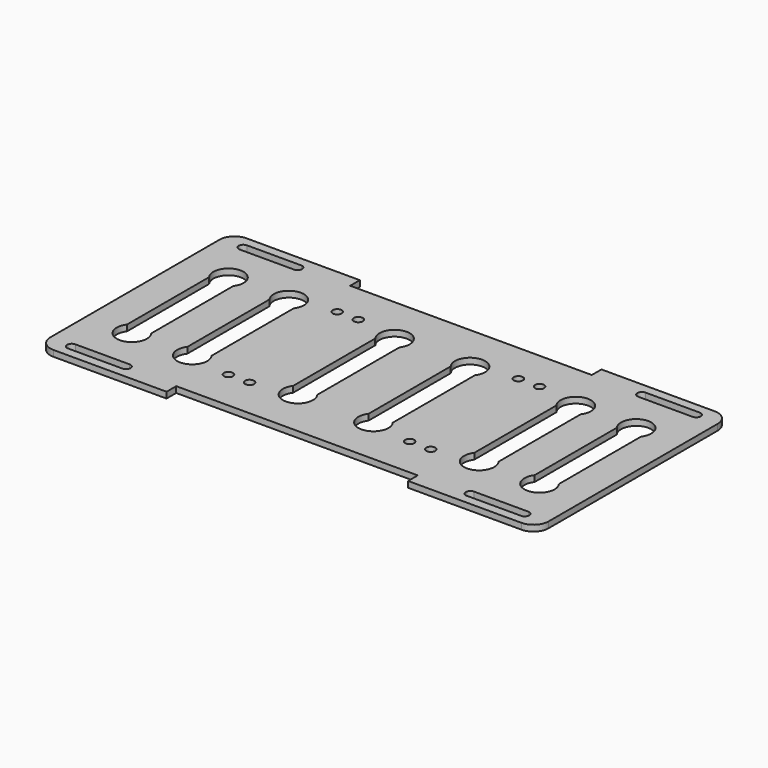
from build123d import *

# Parameters (mm, degrees)
F0_W      = 165
F0_H      = 80
F1_DEPTH  = 2
F2_W      = 21
F2_H      = 3
F3_DEPTH  = 2
F4_R      = 1.49999
F5_W      = 165
F5_H      = 80
F5_R      = 1.5
F6_DEPTH  = 2
F7_DEPTH  = 2
F8_R      = 5
F9_R      = 5
F11_DEPTH = 2.001
F12_W     = 80
F12_H     = 8
F13_DEPTH = 2.001


# Not quite as in the source:
# - a fillet or chamfer is up to 0.001 mm smaller than in the source, because OpenCascade refuses the exact size
# - ends of sketch curves that miss each other by under 0.0002 mm in the source are joined


with BuildPart() as f1:
    # F0 (on Top) → F1 (new body)
    with BuildSketch(Plane.XY):
        Rectangle(F0_W, F0_H)
    extrude(amount=F1_DEPTH)

    # F2 (on face) → F3 (cut)
    with BuildSketch(Plane.XY.offset(2)):
        with Locations((-66, 35.5)):
            Rectangle(F2_W, F2_H)
        with Locations((66, 35.5)):
            Rectangle(F2_W, F2_H)
        with Locations((66, -35.5)):
            Rectangle(F2_W, F2_H)
        with Locations((-66, -35.5)):
            Rectangle(F2_W, F2_H)
    extrude(amount=-F3_DEPTH, mode=Mode.SUBTRACT)

    # F4 (radius 1.5 in the source; OpenCascade refuses exactly that, so slightly less here)
    f4_edges = [f1.edges().sort_by_distance(p)[0] for p in [
        (76.5, -37, 1),
        (-55.5, 34, 1),
        (-55.5, -37, 1),
        (76.5, 34, 1),
        (55.5, 37, 1),
        (55.5, -34, 1),
        (-76.5, -34, 1),
        (-76.5, 37, 1),
        (-76.5, 34, 1),
        (-55.5, 37, 1),
        (76.5, 37, 1),
        (55.5, 34, 1),
        (76.5, -34, 1),
        (55.5, -37, 1),
        (-76.5, -37, 1),
        (-55.5, -34, 1),
    ]]
    fillet(f4_edges, radius=F4_R)

    # F5 (on face) → F6 (join)
    with BuildSketch(Plane.XY.offset(2)):
        Rectangle(F5_W, F5_H)
        with BuildLine():
            ThreePointArc((-76.5, -35.49999), (-76.0606631007, -34.4393368993), (-75.00001, -34))
            Line((-75.00001, -34), (-56.99999, -34))
            ThreePointArc((-56.99999, -34), (-55.9393368993, -34.4393368993), (-55.5, -35.49999))
            ThreePointArc((-55.5, -35.49999), (-55.9393368993, -36.5606631007), (-56.99999, -37))
            Line((-56.99999, -37), (-75.00001, -37))
            ThreePointArc((-75.00001, -37), (-76.0606631007, -36.5606631007), (-76.5, -35.49999))
        make_face(mode=Mode.SUBTRACT)
        with Locations((-33.5, -22.5)):
            Circle(F5_R, mode=Mode.SUBTRACT)
        with Locations((-26.5, -22.5)):
            Circle(F5_R, mode=Mode.SUBTRACT)
        with Locations((26.5, -22.5)):
            Circle(F5_R, mode=Mode.SUBTRACT)
        with Locations((33.5, -22.5)):
            Circle(F5_R, mode=Mode.SUBTRACT)
        with BuildLine():
            ThreePointArc((55.5, -35.49999), (55.9393368993, -34.4393368993), (56.99999, -34))
            Line((56.99999, -34), (75.00001, -34))
            ThreePointArc((75.00001, -34), (76.0606631007, -34.4393368993), (76.5, -35.49999))
            ThreePointArc((76.5, -35.49999), (76.0606631007, -36.5606631007), (75.00001, -37))
            Line((75.00001, -37), (56.99999, -37))
            ThreePointArc((56.99999, -37), (55.9393368993, -36.5606631007), (55.5, -35.49999))
        make_face(mode=Mode.SUBTRACT)
        with BuildLine():
            ThreePointArc((-76.5, 35.50001), (-76.0606631007, 36.5606631007), (-75.00001, 37))
            Line((-75.00001, 37), (-56.99999, 37))
            ThreePointArc((-56.99999, 37), (-55.9393368993, 36.5606631007), (-55.5, 35.50001))
            ThreePointArc((-55.5, 35.50001), (-55.9393368993, 34.4393368993), (-56.99999, 34))
            Line((-56.99999, 34), (-75.00001, 34))
            ThreePointArc((-75.00001, 34), (-76.0606631007, 34.4393368993), (-76.5, 35.50001))
        make_face(mode=Mode.SUBTRACT)
        with Locations((-33.5, 22.5)):
            Circle(F5_R, mode=Mode.SUBTRACT)
        with Locations((-26.5, 22.5)):
            Circle(F5_R, mode=Mode.SUBTRACT)
        with Locations((26.5, 22.5)):
            Circle(F5_R, mode=Mode.SUBTRACT)
        with Locations((33.5, 22.5)):
            Circle(F5_R, mode=Mode.SUBTRACT)
        with BuildLine():
            ThreePointArc((55.5, 35.50001), (55.9393368993, 36.5606631007), (56.99999, 37))
            Line((56.99999, 37), (75.00001, 37))
            ThreePointArc((75.00001, 37), (76.0606631007, 36.5606631007), (76.5, 35.50001))
            ThreePointArc((76.5, 35.50001), (76.0606631007, 34.4393368993), (75.00001, 34))
            Line((75.00001, 34), (56.99999, 34))
            ThreePointArc((56.99999, 34), (55.9393368993, 34.4393368993), (55.5, 35.50001))
        make_face(mode=Mode.SUBTRACT)
    extrude(amount=F6_DEPTH)

    # F7 (cut): a face of the model
    f7_faces = [f1.faces().sort_by_distance(p)[0] for p in [
        (0, 0, 0),
    ]]
    extrude(f7_faces, amount=-F7_DEPTH, mode=Mode.SUBTRACT)

    # F8
    f8_edges = [f1.edges().sort_by_distance(p)[0] for p in [
        (82.5, 40, 3),
    ]]
    fillet(f8_edges, radius=F8_R)

    # F9
    f9_edges = [f1.edges().sort_by_distance(p)[0] for p in [
        (82.5, -40, 3),
        (-82.5, -40, 3),
        (-82.5, 40, 3),
    ]]
    fillet(f9_edges, radius=F9_R)

    # F10 (on face) → F11 (cut, through all)
    with BuildSketch(Plane.XY.offset(4)):
        with BuildLine():
            ThreePointArc((-63.5, 17), (-67.5, 15), (-71.5, 17))
            Line((-71.5, 17), (-71.5, -6.31e-08))
            ThreePointArc((-71.5, -6.31e-08), (-67.5000000315, 4), (-63.5, 0))
            Line((-63.5, 0), (-63.5, 17))
        make_face()
        with BuildLine():
            ThreePointArc((-63.5, 0), (-67.4999999685, -4), (-71.5, -6.31e-08))
            Line((-71.5, -6.31e-08), (-71.5, -17))
            ThreePointArc((-71.5, -17), (-67.5, -15), (-63.5, -17))
            Line((-63.5, -17), (-63.5, 0))
        make_face()
        with BuildLine():
            Line((-71.5, -20), (-71.5, -17))
            ThreePointArc((-71.5, -17), (-69.0811388301, -24.7434164903), (-62.5, -20))
            ThreePointArc((-62.5, -20), (-62.7565835097, -18.4188611699), (-63.5, -17))
            Line((-63.5, -17), (-63.5, -20))
            Line((-63.5, -20), (-71.5, -20))
        make_face()
        with BuildLine():
            ThreePointArc((-63.5, -17), (-67.5, -15), (-71.5, -17))
            Line((-71.5, -17), (-71.5, -20))
            Line((-71.5, -20), (-63.5, -20))
            Line((-63.5, -20), (-63.5, -17))
        make_face()
        with BuildLine():
            ThreePointArc((-63.5, 0), (-67.5000000315, 4), (-71.5, -6.31e-08))
            ThreePointArc((-71.5, -6.31e-08), (-67.4999999685, -4), (-63.5, 0))
        make_face()
        with BuildLine():
            Line((-71.5, 20), (-71.5, 17))
            ThreePointArc((-71.5, 17), (-67.5, 15), (-63.5, 17))
            Line((-63.5, 17), (-63.5, 20))
            Line((-63.5, 20), (-71.5, 20))
        make_face()
        with BuildLine():
            ThreePointArc((-63.5, 17), (-62.7565835097, 18.4188611699), (-62.5, 20))
            ThreePointArc((-62.5, 20), (-69.0811388301, 24.7434164903), (-71.5, 17))
            Line((-71.5, 17), (-71.5, 20))
            Line((-71.5, 20), (-63.5, 20))
            Line((-63.5, 20), (-63.5, 17))
        make_face()
        with BuildLine():
            ThreePointArc((-43.5, 17), (-42.7565835097, 18.4188611699), (-42.5, 20))
            ThreePointArc((-42.5, 20), (-49.0811388301, 24.7434164903), (-51.5, 17))
            Line((-51.5, 17), (-51.5, 20))
            Line((-51.5, 20), (-43.5, 20))
            Line((-43.5, 20), (-43.5, 17))
        make_face()
        with BuildLine():
            Line((-51.5, 20), (-51.5, 17))
            ThreePointArc((-51.5, 17), (-47.5, 15), (-43.5, 17))
            Line((-43.5, 17), (-43.5, 20))
            Line((-43.5, 20), (-51.5, 20))
        make_face()
        with BuildLine():
            ThreePointArc((-43.5, 17), (-47.5, 15), (-51.5, 17))
            Line((-51.5, 17), (-51.5, -2.04e-08))
            ThreePointArc((-51.5, -2.04e-08), (-47.5000000102, 4), (-43.5, 0))
            Line((-43.5, 0), (-43.5, 17))
        make_face()
        with BuildLine():
            ThreePointArc((-43.5, 0), (-47.5000000102, 4), (-51.5, -2.04e-08))
            ThreePointArc((-51.5, -2.04e-08), (-47.4999999898, -4), (-43.5, 0))
        make_face()
        with BuildLine():
            ThreePointArc((-43.5, 0), (-47.4999999898, -4), (-51.5, -2.04e-08))
            Line((-51.5, -2.04e-08), (-51.5, -17))
            ThreePointArc((-51.5, -17), (-47.5, -15), (-43.5, -17))
            Line((-43.5, -17), (-43.5, 0))
        make_face()
        with BuildLine():
            ThreePointArc((-43.5, -17), (-47.5, -15), (-51.5, -17))
            Line((-51.5, -17), (-51.5, -20))
            Line((-51.5, -20), (-43.5, -20))
            Line((-43.5, -20), (-43.5, -17))
        make_face()
        with BuildLine():
            Line((-51.5, -20), (-51.5, -17))
            ThreePointArc((-51.5, -17), (-49.0811388301, -24.7434164903), (-42.5, -20))
            ThreePointArc((-42.5, -20), (-42.7565835097, -18.4188611699), (-43.5, -17))
            Line((-43.5, -17), (-43.5, -20))
            Line((-43.5, -20), (-51.5, -20))
        make_face()
        with BuildLine():
            ThreePointArc((-8.5, 17), (-7.7565835097, 18.4188611699), (-7.5, 20))
            ThreePointArc((-7.5, 20), (-14.0811388301, 24.7434164903), (-16.5, 17))
            Line((-16.5, 17), (-16.5, 20))
            Line((-16.5, 20), (-8.5, 20))
            Line((-8.5, 20), (-8.5, 17))
        make_face()
        with BuildLine():
            Line((-16.5, 20), (-16.5, 17))
            ThreePointArc((-16.5, 17), (-12.5, 15), (-8.5, 17))
            Line((-8.5, 17), (-8.5, 20))
            Line((-8.5, 20), (-16.5, 20))
        make_face()
        with BuildLine():
            ThreePointArc((-8.5, 17), (-12.5, 15), (-16.5, 17))
            Line((-16.5, 17), (-16.5, 8.4e-09))
            ThreePointArc((-16.5, 8.4e-09), (-12.4999999958, 4), (-8.5, 0))
            Line((-8.5, 0), (-8.5, 17))
        make_face()
        with BuildLine():
            ThreePointArc((-8.5, 0), (-12.4999999958, 4), (-16.5, 8.4e-09))
            ThreePointArc((-16.5, 8.4e-09), (-12.5000000042, -4), (-8.5, 0))
        make_face()
        with BuildLine():
            ThreePointArc((-8.5, 0), (-12.5000000042, -4), (-16.5, 8.4e-09))
            Line((-16.5, 8.4e-09), (-16.5, -17))
            ThreePointArc((-16.5, -17), (-12.5, -15), (-8.5, -17))
            Line((-8.5, -17), (-8.5, 0))
        make_face()
        with BuildLine():
            ThreePointArc((-8.5, -17), (-12.5, -15), (-16.5, -17))
            Line((-16.5, -17), (-16.5, -20))
            Line((-16.5, -20), (-8.5, -20))
            Line((-8.5, -20), (-8.5, -17))
        make_face()
        with BuildLine():
            Line((-16.5, -20), (-16.5, -17))
            ThreePointArc((-16.5, -17), (-14.0811388301, -24.7434164903), (-7.5, -20))
            ThreePointArc((-7.5, -20), (-7.7565835097, -18.4188611699), (-8.5, -17))
            Line((-8.5, -17), (-8.5, -20))
            Line((-8.5, -20), (-16.5, -20))
        make_face()
        with BuildLine():
            ThreePointArc((16.5, 17), (17.2434164903, 18.4188611699), (17.5, 20))
            ThreePointArc((17.5, 20), (10.9188611699, 24.7434164903), (8.5, 17))
            Line((8.5, 17), (8.5, 20))
            Line((8.5, 20), (16.5, 20))
            Line((16.5, 20), (16.5, 17))
        make_face()
        with BuildLine():
            Line((8.5, 20), (8.5, 17))
            ThreePointArc((8.5, 17), (12.5, 15), (16.5, 17))
            Line((16.5, 17), (16.5, 20))
            Line((16.5, 20), (8.5, 20))
        make_face()
        with BuildLine():
            ThreePointArc((16.5, 17), (12.5, 15), (8.5, 17))
            Line((8.5, 17), (8.5, 8.4e-09))
            ThreePointArc((8.5, 8.4e-09), (12.5000000042, 4), (16.5, 0))
            Line((16.5, 0), (16.5, 17))
        make_face()
        with BuildLine():
            ThreePointArc((16.5, 0), (12.5000000042, 4), (8.5, 8.4e-09))
            ThreePointArc((8.5, 8.4e-09), (12.4999999958, -4), (16.5, 0))
        make_face()
        with BuildLine():
            ThreePointArc((16.5, 0), (12.4999999958, -4), (8.5, 8.4e-09))
            Line((8.5, 8.4e-09), (8.5, -17))
            ThreePointArc((8.5, -17), (12.5, -15), (16.5, -17))
            Line((16.5, -17), (16.5, 0))
        make_face()
        with BuildLine():
            ThreePointArc((16.5, -17), (12.5, -15), (8.5, -17))
            Line((8.5, -17), (8.5, -20))
            Line((8.5, -20), (16.5, -20))
            Line((16.5, -20), (16.5, -17))
        make_face()
        with BuildLine():
            Line((8.5, -20), (8.5, -17))
            ThreePointArc((8.5, -17), (10.9188611699, -24.7434164903), (17.5, -20))
            ThreePointArc((17.5, -20), (17.2434164903, -18.4188611699), (16.5, -17))
            Line((16.5, -17), (16.5, -20))
            Line((16.5, -20), (8.5, -20))
        make_face()
        with BuildLine():
            ThreePointArc((51.5, 17), (52.2434164903, 18.4188611699), (52.5, 20))
            ThreePointArc((52.5, 20), (45.9188611699, 24.7434164903), (43.5, 17))
            Line((43.5, 17), (43.5, 20))
            Line((43.5, 20), (51.5, 20))
            Line((51.5, 20), (51.5, 17))
        make_face()
        with BuildLine():
            Line((43.5, 20), (43.5, 17))
            ThreePointArc((43.5, 17), (47.5, 15), (51.5, 17))
            Line((51.5, 17), (51.5, 20))
            Line((51.5, 20), (43.5, 20))
        make_face()
        with BuildLine():
            ThreePointArc((51.5, 17), (47.5, 15), (43.5, 17))
            Line((43.5, 17), (43.5, -2.04e-08))
            ThreePointArc((43.5, -2.04e-08), (47.4999999898, 4), (51.5, 0))
            Line((51.5, 0), (51.5, 17))
        make_face()
        with BuildLine():
            ThreePointArc((51.5, 0), (47.4999999898, 4), (43.5, -2.04e-08))
            ThreePointArc((43.5, -2.04e-08), (47.5000000102, -4), (51.5, 0))
        make_face()
        with BuildLine():
            ThreePointArc((51.5, 0), (47.5000000102, -4), (43.5, -2.04e-08))
            Line((43.5, -2.04e-08), (43.5, -17))
            ThreePointArc((43.5, -17), (47.5, -15), (51.5, -17))
            Line((51.5, -17), (51.5, 0))
        make_face()
        with BuildLine():
            ThreePointArc((51.5, -17), (47.5, -15), (43.5, -17))
            Line((43.5, -17), (43.5, -20))
            Line((43.5, -20), (51.5, -20))
            Line((51.5, -20), (51.5, -17))
        make_face()
        with BuildLine():
            Line((43.5, -20), (43.5, -17))
            ThreePointArc((43.5, -17), (45.9188611699, -24.7434164903), (52.5, -20))
            ThreePointArc((52.5, -20), (52.2434164903, -18.4188611699), (51.5, -17))
            Line((51.5, -17), (51.5, -20))
            Line((51.5, -20), (43.5, -20))
        make_face()
        with BuildLine():
            ThreePointArc((71.5, 17), (72.2434164903, 18.4188611699), (72.5, 20))
            ThreePointArc((72.5, 20), (65.9188611699, 24.7434164903), (63.5, 17))
            Line((63.5, 17), (63.5, 20))
            Line((63.5, 20), (71.5, 20))
            Line((71.5, 20), (71.5, 17))
        make_face()
        with BuildLine():
            Line((63.5, 20), (63.5, 17))
            ThreePointArc((63.5, 17), (67.5, 15), (71.5, 17))
            Line((71.5, 17), (71.5, 20))
            Line((71.5, 20), (63.5, 20))
        make_face()
        with BuildLine():
            ThreePointArc((71.5, 17), (67.5, 15), (63.5, 17))
            Line((63.5, 17), (63.5, -2.04e-08))
            ThreePointArc((63.5, -2.04e-08), (67.4999999898, 4), (71.5, 0))
            Line((71.5, 0), (71.5, 17))
        make_face()
        with BuildLine():
            ThreePointArc((71.5, 0), (67.4999999898, 4), (63.5, -2.04e-08))
            ThreePointArc((63.5, -2.04e-08), (67.5000000102, -4), (71.5, 0))
        make_face()
        with BuildLine():
            ThreePointArc((71.5, 0), (67.5000000102, -4), (63.5, -2.04e-08))
            Line((63.5, -2.04e-08), (63.5, -17))
            ThreePointArc((63.5, -17), (67.5, -15), (71.5, -17))
            Line((71.5, -17), (71.5, 0))
        make_face()
        with BuildLine():
            ThreePointArc((71.5, -17), (67.5, -15), (63.5, -17))
            Line((63.5, -17), (63.5, -20))
            Line((63.5, -20), (71.5, -20))
            Line((71.5, -20), (71.5, -17))
        make_face()
        with BuildLine():
            Line((63.5, -20), (63.5, -17))
            ThreePointArc((63.5, -17), (65.9188611699, -24.7434164903), (72.5, -20))
            ThreePointArc((72.5, -20), (72.2434164903, -18.4188611699), (71.5, -17))
            Line((71.5, -17), (71.5, -20))
            Line((71.5, -20), (63.5, -20))
        make_face()
    extrude(amount=-F11_DEPTH, mode=Mode.SUBTRACT)

    # F12 (on face) → F13 (cut, through all)
    with BuildSketch(Plane.XY.offset(4)):
        with Locations((0, -40)):
            Rectangle(F12_W, F12_H)
        with Locations((0, 40)):
            Rectangle(F12_W, F12_H)
    extrude(amount=-F13_DEPTH, mode=Mode.SUBTRACT)


solid = f1.part
